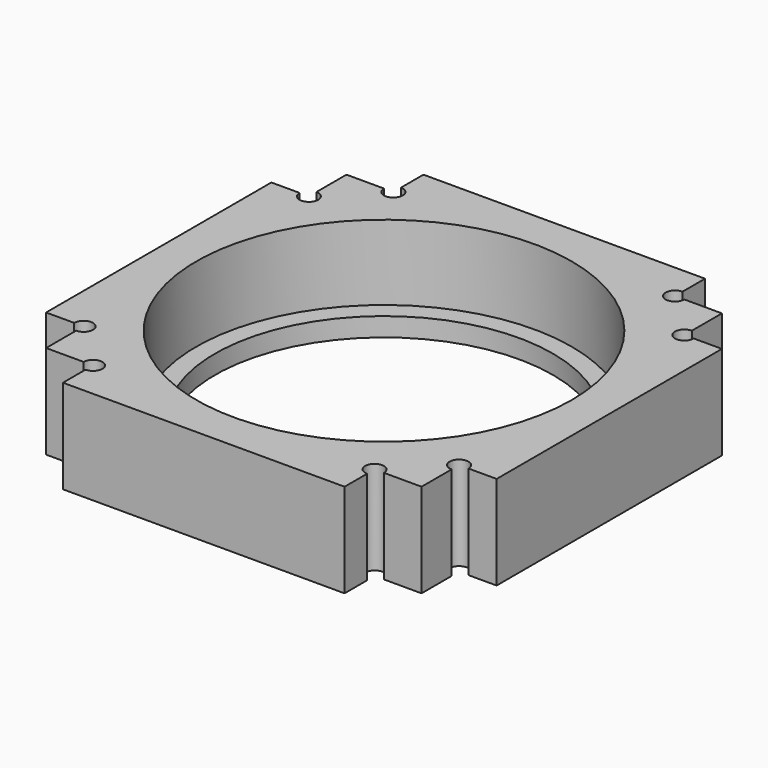
from build123d import *

# Parameters (mm, degrees)
F0_R            = 14.2875
F1_DEPTH        = 7.9375
F2_R            = 15.875
F3_DEPTH        = 6.35
F4_R            = 0.79375
F5_DEPTH        = 7.9375
F5_COPIES_COUNT = 4


# Not quite as in the source:
# - a pattern or mirror of a feature is missing from the dataset's text; its kind, count and spacing are read off the source's solid


with BuildPart() as f1:
    # F0 (on Top) → F1 (new body)
    with BuildSketch(Plane.XY):
        Polygon((19.05, 11.90625), (15.875, 11.90625), (15.875, 15.875), (11.90625, 15.875), (11.90625, 19.05), (-11.90625, 19.05), (-11.90625, 15.875), (-15.875, 15.875), (-15.875, 11.90625), (-19.05, 11.90625), (-19.05, -11.90625), (-15.875, -11.90625), (-15.875, -15.875), (-11.90625, -15.875), (-11.90625, -19.05), (11.90625, -19.05), (11.90625, -15.875), (15.875, -15.875), (15.875, -11.90625), (19.05, -11.90625), align=None)
        Circle(F0_R, mode=Mode.SUBTRACT)
    extrude(amount=F1_DEPTH)

    # F2 (on face) → F3 (cut)
    with BuildSketch(Plane.XY.offset(7.9375)):
        Circle(F2_R)
    extrude(amount=-F3_DEPTH, mode=Mode.SUBTRACT)

    # F4 (on face) → F5 (cut, through all)
    with BuildSketch(Plane.XY.offset(7.9375)):
        with Locations((11.90625, 15.875)):
            Circle(F4_R)
        with Locations((-11.90625, 15.875)):
            Circle(F4_R)
    f5 = extrude(amount=-F5_DEPTH, mode=Mode.SUBTRACT)

    # F5_copies: F5 ×4 about axis
    f5_copies_axis = Axis((0, 0, 0), (0, 0, 1))
    for i in range(1, F5_COPIES_COUNT):
        add(f5.rotate(f5_copies_axis, i * 360 / F5_COPIES_COUNT), mode=Mode.SUBTRACT)


solid = f1.part
